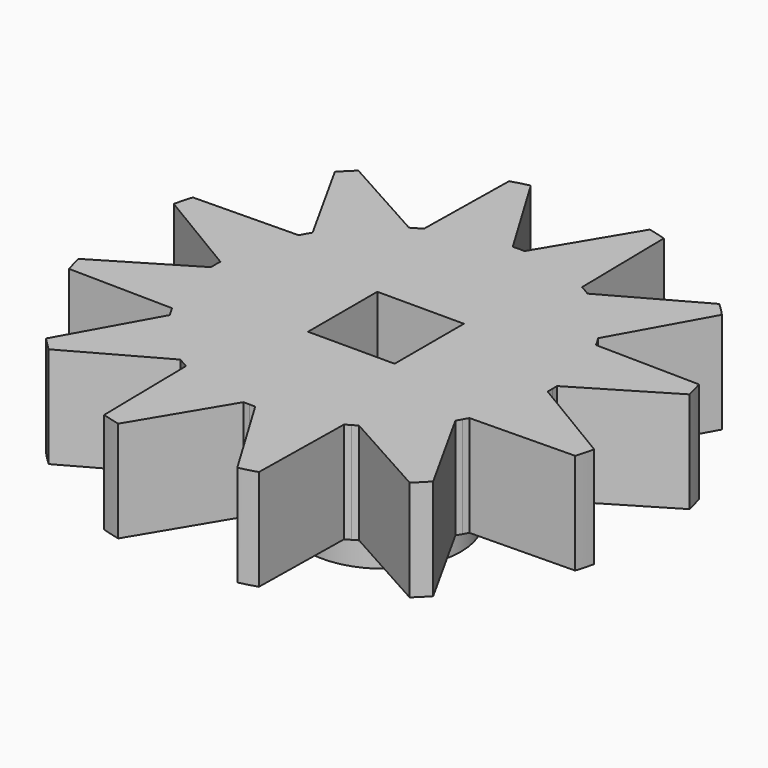
from build123d import *

# Parameters (mm, degrees)
F0_R            = 11
F1_DEPTH        = 4.2
F3_DEPTH        = 4.201
F3_COPIES_COUNT = 12
F5_R            = 3.2
F6_DEPTH        = 3
F7_W            = 3.6
F7_H            = 3.6
F8_DEPTH        = 7.201


# Not quite as in the source:
# - a pattern or mirror of a feature is missing from the dataset's text; its kind, count and spacing are read off the source's solid


with BuildPart() as f1:
    # F0 (on Top) → F1 (new body)
    with BuildSketch(Plane.XY):
        Circle(F0_R)
    extrude(amount=F1_DEPTH)

    # F2 (on face) → F3 (cut, through all)
    with BuildSketch(Plane(origin=(0, 0, 0), x_dir=(1, 0, 0), z_dir=(0, 0, -1))):
        with BuildLine():
            ThreePointArc((6.9957357891, 0.2442964769), (6.9989338661, 0.1221668451), (7, 0))
            Line((7, 0), (8.3441911265, 0))
            Line((8.3441911265, 0), (11, 0))
            ThreePointArc((11, 0), (10.9292904124, 1.2452353514), (10.7180707126, 2.4744615978))
            Line((10.7180707126, 2.4744615978), (6.9957357891, 0.2442964769))
        make_face()
        with BuildLine():
            Line((8.3441911265, 0), (7, 0))
            Line((7, 0), (6.9957357891, -0.2442964769))
            Line((6.9957357891, -0.2442964769), (10.7180707126, -2.4744615978))
            ThreePointArc((10.7180707126, -2.4744615978), (10.9292904124, -1.2452353514), (11, 0))
            Line((11, 0), (8.3441911265, 0))
        make_face()
    f3 = extrude(amount=-F3_DEPTH, mode=Mode.SUBTRACT)

    # F3_copies: F3 ×12 about axis
    f3_copies_axis = Axis((0, 0, 0), (0, 0, 1))
    for i in range(1, F3_COPIES_COUNT):
        add(f3.rotate(f3_copies_axis, i * 360 / F3_COPIES_COUNT), mode=Mode.SUBTRACT)

    # F5 (on face) → F6 (join)
    with BuildSketch(Plane(origin=(0, 0, 0), x_dir=(1, 0, 0), z_dir=(0, 0, -1))):
        with Locations((-0.0057600341, -0.0028142263)):
            Circle(F5_R)
    extrude(amount=F6_DEPTH)

    # F7 (on face) → F8 (cut, through all)
    with BuildSketch(Plane(origin=(0, 0, -3), x_dir=(1, 0, 0), z_dir=(0, 0, -1))):
        with Locations((0.0985847846, 0.0223461993)):
            Rectangle(F7_W, F7_H)
    extrude(amount=-F8_DEPTH, mode=Mode.SUBTRACT)


solid = f1.part
